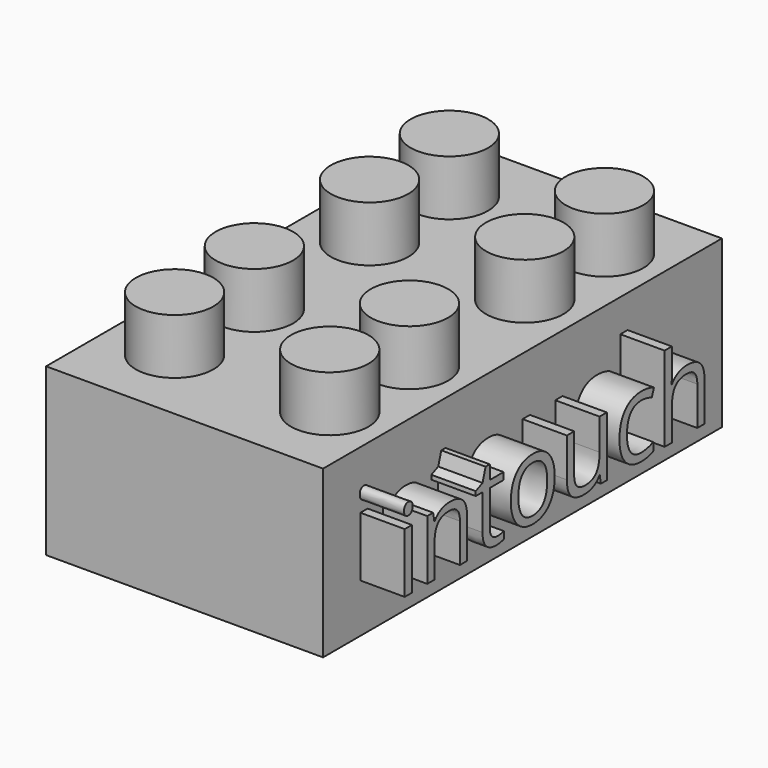
from build123d import *

# Parameters (mm, degrees)
F0_W         = 25
F0_H         = 45
F1_DEPTH     = 15
F2_R         = 3.5
F3_DEPTH     = 5
F5_TEXT_SIZE = 10.0654562832
F6_DEPTH     = 4


# Not quite as in the source:
# - Text() gives the source's letters only with a copy of the font that has no kerning and outlines rounded to 1/6400 em; it was checked with that copy


with BuildPart() as f1:
    # F0 (on Top) → F1 (new body)
    with BuildSketch(Plane.XY):
        with Locations((-0.675675348, 3.9295725853)):
            Rectangle(F0_W, F0_H)
    extrude(amount=F1_DEPTH)

    # F2 (on face) → F3 (join)
    with BuildSketch(Plane.XY.offset(15)):
        with Locations((-7.175675348, 19.4295725853)):
            Circle(F2_R)
        with Locations((-7.175675348, 10.4295725853)):
            Circle(F2_R)
        with Locations((6.824324652, 10.4295725853)):
            Circle(F2_R)
        with Locations((6.824324652, 19.4295725853)):
            Circle(F2_R)
        with Locations((6.824324652, -2.5704274147)):
            Circle(F2_R)
        with Locations((6.824324652, -11.5704274147)):
            Circle(F2_R)
        with Locations((-7.175675348, -11.5704274147)):
            Circle(F2_R)
        with Locations((-7.175675348, -2.5704274147)):
            Circle(F2_R)
    extrude(amount=F3_DEPTH)

    # F5 (on face) → F6 (join)
    with BuildSketch(Plane.YZ.offset(11.824324652)):
        with Locations((-15.2258328162, 4.3970439583)):
            Text('intouch', F5_TEXT_SIZE, font='Open Sans', text_align=(TextAlign.LEFT, TextAlign.BOTTOM))
    extrude(amount=F6_DEPTH)


solid = f1.part
